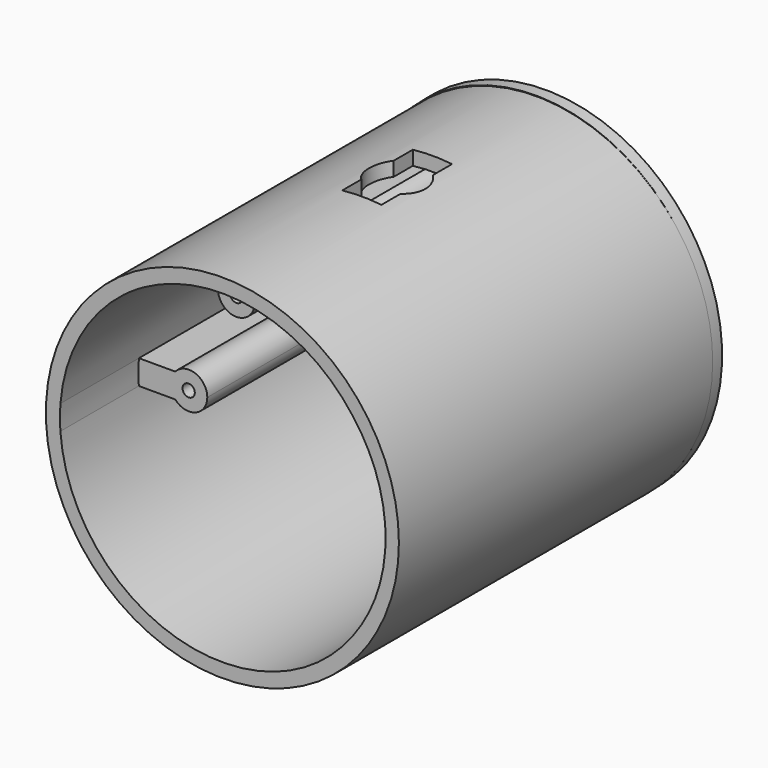
from build123d import *

# Parameters (mm, degrees)
F0_R     = 14.4
F1_DEPTH = 8
F0_R_2   = 0.5
F2_DEPTH = 24
F4_DEPTH = 25
F5_R     = 14.4
F6_DEPTH = 1


# Not quite as in the source:
# - a feature names something its author has since deleted; it is built from what else it names


with BuildPart() as f1:
    # F0 (on Front) → F1 (new body)
    with BuildSketch(Plane.XZ):
        with Locations((0.0303304768, -0.0397499959)):
            Circle(F0_R)
        with BuildLine():
            ThreePointArc((10.6755009314, 7.8496635433), (12.4816793636, 4.6139026446), (13.301518859, 1))
            ThreePointArc((13.301518859, 1), (13.3431044371, 0.0001181292), (13.3076524455, -1))
            ThreePointArc((13.3076524455, -1), (12.4958940048, -4.6561546149), (10.6755009314, -7.9291635352))
            ThreePointArc((10.6755009314, -7.9291635352), (-3.6648740835, -12.7640559989), (-13.1848282407, -1))
            ThreePointArc((-13.1848282407, -1), (-13.2196095565, 0.0001136945), (-13.1788110527, 1))
            ThreePointArc((-13.1788110527, 1), (-11.605380035, 6.2984469785), (-8.0072458781, 10.4939989255))
            ThreePointArc((-8.0072458781, 10.4939989255), (-7.1861367371, 11.0726350293), (-6.3235511773, 11.5874030488))
            ThreePointArc((-6.3235511773, 11.5874030488), (2.8757590992, 12.9011168976), (10.6755009314, 7.8496635433))
        make_face(mode=Mode.SUBTRACT)
    extrude(amount=F1_DEPTH)

    # F0 (on Front) → F2 (join)
    with BuildSketch(Plane.XZ):
        with Locations((0.0303304768, -0.0397499959)):
            Circle(F0_R)
        with BuildLine():
            ThreePointArc((10.6755009314, 7.8496635433), (12.4816793636, 4.6139026446), (13.301518859, 1))
            ThreePointArc((13.301518859, 1), (13.3431044371, 0.0001181292), (13.3076524455, -1))
            ThreePointArc((13.3076524455, -1), (12.4958940048, -4.6561546149), (10.6755009314, -7.9291635352))
            ThreePointArc((10.6755009314, -7.9291635352), (-3.6648740835, -12.7640559989), (-13.1848282407, -1))
            ThreePointArc((-13.1848282407, -1), (-13.2196095565, 0.0001136945), (-13.1788110527, 1))
            ThreePointArc((-13.1788110527, 1), (-11.605380035, 6.2984469785), (-8.0072458781, 10.4939989255))
            ThreePointArc((-8.0072458781, 10.4939989255), (-7.1861367371, 11.0726350293), (-6.3235511773, 11.5874030488))
            ThreePointArc((-6.3235511773, 11.5874030488), (2.8757590992, 12.9011168976), (10.6755009314, 7.8496635433))
        make_face(mode=Mode.SUBTRACT)
        with BuildLine():
            ThreePointArc((11.3320508076, -1), (11.5318516526, -0.5176380902), (11.6, 0))
            ThreePointArc((11.6, 0), (11.5318516526, 0.5176380902), (11.3320508076, 1))
            ThreePointArc((11.3320508076, 1), (7.6, 0), (11.3320508076, -1))
        make_face()
        with Locations((9.6801056635, 0)):
            Circle(F0_R_2, mode=Mode.SUBTRACT)
        with BuildLine():
            ThreePointArc((-10.2180339887, 1), (-10.6, 0), (-10.2180339887, -1))
            ThreePointArc((-10.2180339887, -1), (-8.5647668653, -1.4012585384), (-7.6, 0))
            ThreePointArc((-7.6, 0), (-8.5647668653, 1.4012585384), (-10.2180339887, 1))
        make_face()
        with Locations((-9.119440236, 0)):
            Circle(F0_R_2, mode=Mode.SUBTRACT)
        with BuildLine():
            ThreePointArc((-3.7285347361, 8.0512374523), (-4.0895399111, 9.0272962561), (-4.9987891209, 9.5335386876))
            ThreePointArc((-4.9987891209, 9.5335386876), (-6.0454932887, 9.3092433042), (-6.6761302568, 8.4442606176))
            ThreePointArc((-6.6761302568, 8.4442606176), (-5.4267854851, 6.5643962904), (-3.7285347361, 8.0512374523))
        make_face()
        with Locations((-5.2285347361, 8.0512374523)):
            Circle(F0_R_2, mode=Mode.SUBTRACT)
        with BuildLine():
            ThreePointArc((-13.1788110527, 1), (-13.2196095565, 0.0001136945), (-13.1848282407, -1))
            Line((-13.1848282407, -1), (-10.8320508076, -1))
            Line((-10.8320508076, -1), (-10.2180339887, -1))
            ThreePointArc((-10.2180339887, -1), (-10.6, 0), (-10.2180339887, 1))
            Line((-10.2180339887, 1), (-10.8320508076, 1))
            Line((-10.8320508076, 1), (-13.1788110527, 1))
        make_face()
        with BuildLine():
            Line((-4.9987891209, 9.5335386876), (-6.3235511773, 11.5874030488))
            ThreePointArc((-6.3235511773, 11.5874030488), (-7.1861367371, 11.0726350293), (-8.0072458781, 10.4939989255))
            Line((-8.0072458781, 10.4939989255), (-6.6761302568, 8.4442606176))
            ThreePointArc((-6.6761302568, 8.4442606176), (-6.0454932887, 9.3092433042), (-4.9987891209, 9.5335386876))
        make_face()
        with BuildLine():
            ThreePointArc((11.3320508076, 1), (11.5318516526, 0.5176380902), (11.6, 0))
            ThreePointArc((11.6, 0), (11.5318516526, -0.5176380902), (11.3320508076, -1))
            Line((11.3320508076, -1), (13.25, -1))
            Line((13.25, -1), (13.3076524455, -1))
            ThreePointArc((13.3076524455, -1), (13.3431044371, 0.0001181292), (13.301518859, 1))
            Line((13.301518859, 1), (13.25, 1))
            Line((13.25, 1), (11.3320508076, 1))
        make_face()
    extrude(amount=-F2_DEPTH)

    # F3 (on Top) → F4 (cut)
    with BuildSketch(Plane.XY):
        with BuildLine():
            Line((1.6, 6.2556717858), (1.6, 8.2034006216))
            ThreePointArc((1.6, 8.2034006216), (0, 7.5556717858), (-1.6, 8.2034006216))
            Line((-1.6, 8.2034006216), (-1.6, 6.2556717858))
            Line((-1.6, 6.2556717858), (1.6, 6.2556717858))
        make_face()
        with BuildLine():
            ThreePointArc((1.6, 8.2034006216), (2.1177818585, 8.9584538635), (2.3, 9.8556717858))
            ThreePointArc((2.3, 9.8556717858), (2.1177818585, 10.752889708), (1.6, 11.50794295))
            ThreePointArc((1.6, 11.50794295), (0, 12.1556717858), (-1.6, 11.50794295))
            ThreePointArc((-1.6, 11.50794295), (-2.3, 9.8556717858), (-1.6, 8.2034006216))
            ThreePointArc((-1.6, 8.2034006216), (0, 7.5556717858), (1.6, 8.2034006216))
        make_face()
        with BuildLine():
            ThreePointArc((-1.6, 11.50794295), (0, 12.1556717858), (1.6, 11.50794295))
            Line((1.6, 11.50794295), (1.6, 13.4556717858))
            Line((1.6, 13.4556717858), (-1.6, 13.4556717858))
            Line((-1.6, 13.4556717858), (-1.6, 11.50794295))
        make_face()
    extrude(amount=F4_DEPTH, mode=Mode.SUBTRACT)

    # F5 (on face) → F6 (join)
    with BuildSketch(Plane(origin=(0, 24, 0), x_dir=(-1, 0, 0), z_dir=(0, 1, 0))):
        Circle(F5_R)
    extrude(amount=F6_DEPTH)


solid = f1.part
